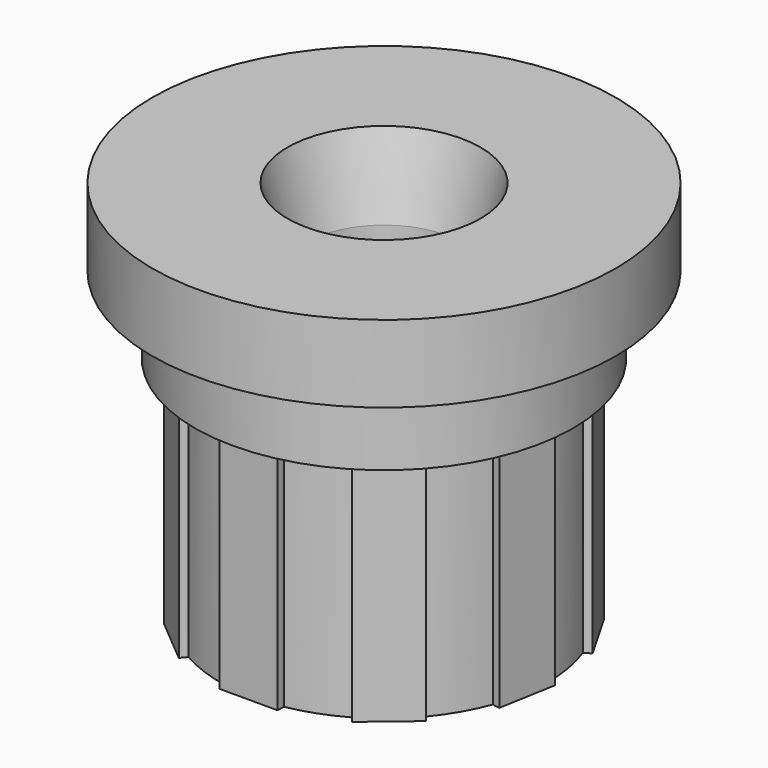
from build123d import *

# Parameters (mm, degrees)
F3_DEPTH        = 6
F3_COPIES_COUNT = 9


# Not quite as in the source:
# - a pattern or mirror of a feature is missing from the dataset's text; its kind, count and spacing are read off the source's solid


with BuildPart() as f1:
    # F0 (on Front) → F1 (revolve)
    with BuildSketch(Plane.XZ):
        Polygon((6, 0), (2.5, 0), (2, -2), (2, -10), (4.25, -10), (4.25, -4), (4.9, -4), (4.9, -2), (6, -2), align=None)
    revolve(axis=Axis((0, 0, -12.1953526796), (0, 0, -1)))

    # F2 (on face) → F3 (join, through all)
    with BuildSketch(Plane(origin=(0, 0, -10), x_dir=(1, 0, 0), z_dir=(0, 0, -1))):
        with BuildLine():
            ThreePointArc((-0.75, 4.1833001327), (0, 4.25), (0.75, 4.1833001327))
            Line((0.75, 4.1833001327), (0.75, 4.3833001327))
            Line((0.75, 4.3833001327), (-0.75, 4.3833001327))
            Line((-0.75, 4.3833001327), (-0.75, 4.1833001327))
        make_face()
    f3 = extrude(amount=-F3_DEPTH)

    # F3_copies: F3 ×9 about axis
    f3_copies_axis = Axis((0, 0, 0), (0, 0, 1))
    for i in range(1, F3_COPIES_COUNT):
        add(f3.rotate(f3_copies_axis, i * 360 / F3_COPIES_COUNT))


solid = f1.part
